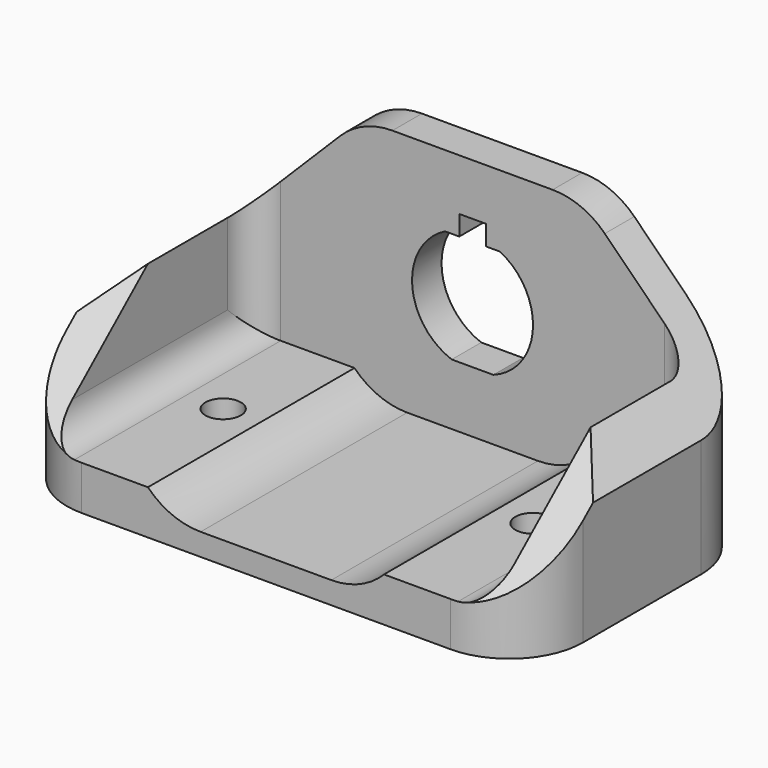
from build123d import *

# Parameters (mm, degrees)
F0_W          = 35
F0_H          = 18
F1_DEPTH      = 20
F2_W          = 30
F2_H          = 23.709095493
F3_DEPTH      = 15
F5_DEPTH      = 32.5
F6_T1_DEPTH   = 53.9336597593
F7_R          = 2
F10_DEPTH     = 25
F11_R         = 5
F12_W         = 16
F12_H         = 17.5
F13_DEPTH     = 1.5
F14_T4_DEPTH  = 26.4267855357
F14_T9_DEPTH  = 26.4267855357
F14_T11_DEPTH = 28
F14_T13_DEPTH = 28
F15_R         = 1.2
F16_DEPTH     = 3.0010001


# Not quite as in the source:
# - a fillet or chamfer that OpenCascade refuses, or shapes differently, is made with other operations: its cross-section is extruded or revolved along the edge and cut away or added


with BuildPart() as f1:
    # F0 (on Front) → F1 (new body)
    with BuildSketch(Plane.XZ):
        with Locations((0, 9)):
            Rectangle(F0_W, F0_H)
    extrude(amount=F1_DEPTH)

    # F2 (on face) → F3 (cut)
    with BuildSketch(Plane.XY.offset(18)):
        with Locations((0, -14.3545477465)):
            Rectangle(F2_W, F2_H)
    extrude(amount=-F3_DEPTH, mode=Mode.SUBTRACT)

    # F4 (on face) → F5 (cut, symmetric)
    with BuildSketch(Plane(origin=(15, 0, 0), x_dir=(0, -1, 0), z_dir=(-1, 0, 0))):
        Polygon((20, 18), (2.5, 18), (20, 3), align=None)
    extrude(amount=F5_DEPTH, both=True, mode=Mode.SUBTRACT)

    # F6: chamfer of 10 on 2 edges, made by hand

    # F6_s2 → F6_t1 (cut)
    with BuildSketch(Plane.XZ.offset(-25.7168298797)):
        Polygon((17.5, 8), (7.5, 18), (17.5, 18), align=None)
        Polygon((-7.5, 18), (-17.5, 8), (-17.5, 18), align=None)
    extrude(amount=F6_T1_DEPTH, mode=Mode.SUBTRACT)

    # F7
    f7_edges = [f1.edges().sort_by_distance(p)[0] for p in [
        (-15, -2.5, 6.75),
        (15, -2.5, 6.75),
        (-15, -11.25, 3),
        (15, -11.25, 3),
    ]]
    fillet(f7_edges, radius=F7_R)

    # F8 (on face) → F10 (cut)
    with BuildSketch(Plane(origin=(0, 0, 0), x_dir=(-1, 0, 0), z_dir=(0, 1, 0))):
        with BuildLine():
            Line((-1.409787218, 5.65), (1.409787218, 5.65))
            ThreePointArc((1.409787218, 5.65), (4.0923866141, 9.2502565294), (1.8674849397, 13.15))
            Line((1.8674849397, 13.15), (0.9, 13.15))
            Line((0.9, 13.15), (0.9, 14.5))
            Line((0.9, 14.5), (-0.9, 14.5))
            Line((-0.9, 14.5), (-0.9, 13.15))
            Line((-0.9, 13.15), (-1.8674849397, 13.15))
            ThreePointArc((-1.8674849397, 13.15), (-4.0923866141, 9.2502565294), (-1.409787218, 5.65))
        make_face()
    extrude(amount=-F10_DEPTH, mode=Mode.SUBTRACT)

    # F11
    f11_edges = [f1.edges().sort_by_distance(p)[0] for p in [
        (7.5, -1.25, 18),
        (-7.5, -1.25, 18),
        (17.5, 0, 4),
        (-17.5, 0, 4),
    ]]
    fillet(f11_edges, radius=F11_R)

    # F12 (on face) → F13 (cut)
    with BuildSketch(Plane.XY.offset(3)):
        with Locations((0, -11.25)):
            Rectangle(F12_W, F12_H)
    extrude(amount=-F13_DEPTH, mode=Mode.SUBTRACT)

    # F14: fillet of radius 5 on 4 edges, made by hand


with BuildPart() as f14_tool2:
    # F14_s3 → F14_t4 (new body)
    with BuildSketch(Plane.XZ.offset(20)):
        with BuildLine():
            ThreePointArc((8, 3), (6.3657774588, 1.8902277714), (4.4292857857, 1.5))
            Line((4.4292857857, 1.5), (8, 1.5))
            Line((8, 1.5), (8, 3))
        make_face()
    extrude(amount=-F14_T4_DEPTH)

    split(bisect_by=Plane.XZ, keep=Keep.TOP)


with BuildPart() as f1_1:
    add(f1.part)

    # F14_t1: union F14_tool2
    add(f14_tool2.part)


with BuildPart() as f14_tool7:
    # F14_s8 → F14_t9 (new body)
    with BuildSketch(Plane.XZ.offset(-6.4267855357)):
        with BuildLine():
            ThreePointArc((-8, 3), (-6.3657774588, 1.8902277714), (-4.4292857857, 1.5))
            Line((-4.4292857857, 1.5), (-8, 1.5))
            Line((-8, 1.5), (-8, 3))
        make_face()
    extrude(amount=F14_T9_DEPTH)

    split(bisect_by=Plane.XZ, keep=Keep.TOP)


with BuildPart() as f1_2:
    add(f1_1.part)

    # F14_t6: union F14_tool7
    add(f14_tool7.part)

    # F14_s12 → F14_t11 (cut)
    with BuildSketch(Plane.XY.offset(-12.5)):
        with BuildLine():
            ThreePointArc((17.5, -15), (16.0355339059, -18.5355339059), (12.5, -20))
            Line((12.5, -20), (17.5, -20))
            Line((17.5, -20), (17.5, -15))
        make_face()
    extrude(amount=F14_T11_DEPTH, mode=Mode.SUBTRACT)

    # F14_s14 → F14_t13 (cut)
    with BuildSketch(Plane.XY.offset(-12.5)):
        with BuildLine():
            ThreePointArc((-17.5, -15), (-16.0355339059, -18.5355339059), (-12.5, -20))
            Line((-12.5, -20), (-17.5, -20))
            Line((-17.5, -20), (-17.5, -15))
        make_face()
    extrude(amount=F14_T13_DEPTH, mode=Mode.SUBTRACT)

    # F15 (on face) → F16 (cut, through all)
    with BuildSketch(Plane.XY.offset(3)):
        with Locations((-10.5, -10.5)):
            Circle(F15_R)
        with BuildLine():
            ThreePointArc((11.7, -10.5), (10.5, -9.3), (9.3, -10.5))
            ThreePointArc((9.3, -10.5), (10.5, -11.7), (11.7, -10.5))
        make_face()
    extrude(amount=-F16_DEPTH, mode=Mode.SUBTRACT)


solid = f1_2.part
